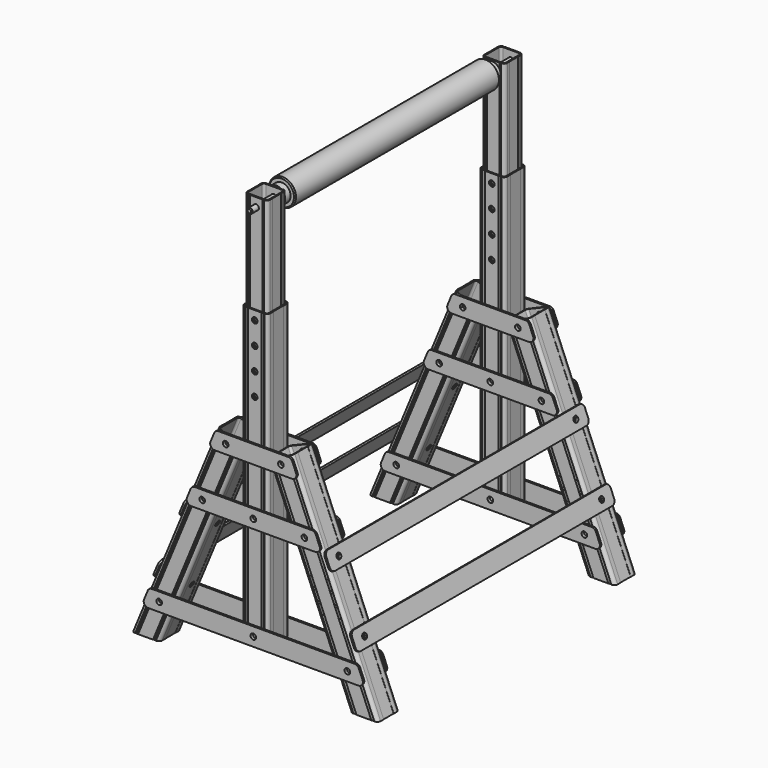
from build123d import *

# Parameters (mm, degrees)
F0_R      = 6.25
F1_DEPTH  = 60
F2_R      = 6.25
F3_DEPTH  = 57.7
F4_R      = 7.5
F6_REACH  = 575.042655099
F7_W      = 57.7
F7_H      = 653.6524637726
F7_R      = 6.25
F8_DEPTH  = 60
F9_R      = 7.5
F11_DEPTH = 653.6524637726
F15_W     = 51
F15_H     = 610
F15_R     = 6.25
F16_DEPTH = 26.15
F17_R     = 7.5
F19_DEPTH = 610
F21_R     = 6.25
F22_DEPTH = 4
F23_R     = 10
F23_2_R   = 10
F23_3_R   = 10
F27_W     = 720
F27_H     = 40
F27_R     = 6.25
F28_DEPTH = 4
F29_R     = 10
F29_2_R   = 10
F32_R     = 5.9
F33_DEPTH = 375
F36_SIZE  = 2
F38_SIZE  = 2.5


# Not quite as in the source:
# - a feature names something its author has since deleted; it is built from what else it names


with BuildPart() as f1:
    # F0 (on Front) → F1 (new body)
    with BuildSketch(Plane.XZ):
        Polygon((-62.4540299569, 0), (0, 0), (-191.3417161825, 461.9397662556), (-244.6495652084, 439.8589322082), align=None)
        with Locations((-64.9222677495, 81.3475362274)):
            Circle(F0_R, mode=Mode.SUBTRACT)
        with Locations((-160.5931258407, 312.3174193552)):
            Circle(F0_R, mode=Mode.SUBTRACT)
        with Locations((-213.0207560747, 438.8889153093)):
            Circle(F0_R, mode=Mode.SUBTRACT)
    extrude(amount=F1_DEPTH)

    # F2 (on face) → F3 (cut, through all)
    with BuildSketch(Plane(origin=(0, 0, 0), x_dir=(0, 1, 0), z_dir=(0.9238795325, 0, 0.3826834324))):
        with Locations((-30, 150)):
            Circle(F2_R)
        with Locations((-30, 300)):
            Circle(F2_R)
    extrude(amount=-F3_DEPTH, mode=Mode.SUBTRACT)

    # F4
    f4_edges = [f1.edges().sort_by_distance(p)[0] for p in [
        (-153.551798, -60, 219.929466),
        (-95.670858, -60, 230.969883),
        (-153.551798, 0, 219.929466),
        (-95.670858, 0, 230.969883),
    ]]
    fillet(f4_edges, radius=F4_R)

    f6_end = f1.faces().sort_by_distance((-31.2270149784, -30, 0))[0]
    # F5 (on face) → F6 (cut, up to a face of the model that its end follows)
    with BuildSketch(Plane(origin=(-191.3417161825, 0, 461.9397662556), x_dir=(0.9238795325, 0, 0.3826834324), z_dir=(-0.3826834324, 0, 0.9238795325))):
        Polygon((-45.2, -59), (-46.2, -60), (-44.2, -60), align=None)
        Polygon((-47.2, -59), (-48.2, -60), (-46.2, -60), align=None)
        Polygon((-49.2, -59), (-50.2, -60), (-48.2, -60), align=None)
        Polygon((-8.5, -59), (-9.5, -60), (-7.5, -60), align=None)
        Polygon((-10.5, -59), (-11.5, -60), (-9.5, -60), align=None)
        Polygon((-12.5, -59), (-13.5, -60), (-11.5, -60), align=None)
        Polygon((-0.3, -44), (0, -44), (0, -16), (-0.3, -16), (-0.3, -30), align=None)
        Polygon((-57.4, -44), (-57.4, -30), (-57.4, -16), (-57.7, -16), (-57.7, -44), align=None)
        Polygon((-48.2, 0), (-50.2, 0), (-49.2, -1), align=None)
        Polygon((-46.2, 0), (-48.2, 0), (-47.2, -1), align=None)
        Polygon((-44.2, 0), (-46.2, 0), (-45.2, -1), align=None)
        Polygon((-7.5, 0), (-9.5, 0), (-8.5, -1), align=None)
        Polygon((-9.5, 0), (-11.5, 0), (-10.5, -1), align=None)
        Polygon((-11.5, 0), (-13.5, 0), (-12.5, -1), align=None)
        with BuildLine():
            Line((-54.8, -30), (-54.8, -52.5))
            ThreePointArc((-54.8, -52.5), (-53.4526911935, -55.7526911935), (-50.2, -57.1))
            Line((-50.2, -57.1), (-28.85, -57.1))
            Line((-28.85, -57.1), (-7.5, -57.1))
            ThreePointArc((-7.5, -57.1), (-4.2473088065, -55.7526911935), (-2.9, -52.5))
            Line((-2.9, -52.5), (-2.9, -30))
            Line((-2.9, -30), (-2.9, -7.5))
            ThreePointArc((-2.9, -7.5), (-4.2473088065, -4.2473088065), (-7.5, -2.9))
            Line((-7.5, -2.9), (-28.85, -2.9))
            Line((-28.85, -2.9), (-50.2, -2.9))
            ThreePointArc((-50.2, -2.9), (-53.4526911935, -4.2473088065), (-54.8, -7.5))
            Line((-54.8, -7.5), (-54.8, -30))
        make_face()
    f6_long = extrude(amount=-F6_REACH, mode=Mode.PRIVATE)
    add(split(f6_long, bisect_by=f6_end, keep=Keep.BOTTOM, mode=Mode.PRIVATE), mode=Mode.SUBTRACT)


with BuildPart() as f8:
    # F7 (on face) → F8 (new body)
    with BuildSketch(Plane.XZ.offset(60)):
        with Locations((-274.4995652084, 393.1737681137)):
            Rectangle(F7_W, F7_H)
        with Locations((-274.4995652084, 81.3475362274)):
            Circle(F7_R, mode=Mode.SUBTRACT)
        with Locations((-274.4995652084, 312.3174193552)):
            Circle(F7_R, mode=Mode.SUBTRACT)
        with Locations((-274.4995652084, 600)):
            Circle(F7_R, mode=Mode.SUBTRACT)
        with Locations((-274.4995652084, 650)):
            Circle(F7_R, mode=Mode.SUBTRACT)
        with Locations((-274.4995652084, 700)):
            Circle(F7_R, mode=Mode.SUBTRACT)
        with Locations((-274.4995652084, 550)):
            Circle(F7_R, mode=Mode.SUBTRACT)
    extrude(amount=-F8_DEPTH)

    # F9
    f9_edges = [f8.edges().sort_by_distance(p)[0] for p in [
        (-303.349565, 0, 393.173768),
        (-303.349565, -60, 393.173768),
        (-245.649565, -60, 393.173768),
        (-245.649565, 0, 393.173768),
    ]]
    fillet(f9_edges, radius=F9_R)

    # F10 (on face) → F11 (cut, through all)
    with BuildSketch(Plane.XY.offset(720)):
        Polygon((-290.8495652084, -59), (-291.8495652084, -60), (-289.8495652084, -60), align=None)
        Polygon((-292.8495652084, -59), (-293.8495652084, -60), (-291.8495652084, -60), align=None)
        Polygon((-294.8495652084, -59), (-295.8495652084, -60), (-293.8495652084, -60), align=None)
        Polygon((-303.3495652084, -16), (-303.3495652084, -44), (-303.0495652084, -44), (-303.0495652084, -30), (-303.0495652084, -16), align=None)
        Polygon((-254.1495652084, -59), (-255.1495652084, -60), (-253.1495652084, -60), align=None)
        Polygon((-256.1495652084, -59), (-257.1495652084, -60), (-255.1495652084, -60), align=None)
        Polygon((-258.1495652084, -59), (-259.1495652084, -60), (-257.1495652084, -60), align=None)
        Polygon((-245.9495652084, -44), (-245.6495652084, -44), (-245.6495652084, -16), (-245.9495652084, -16), (-245.9495652084, -30), align=None)
        Polygon((-253.1495652084, 0), (-255.1495652084, 0), (-254.1495652084, -1), align=None)
        Polygon((-255.1495652084, 0), (-257.1495652084, 0), (-256.1495652084, -1), align=None)
        Polygon((-257.1495652084, 0), (-259.1495652084, 0), (-258.1495652084, -1), align=None)
        Polygon((-293.8495652084, 0), (-295.8495652084, 0), (-294.8495652084, -1), align=None)
        Polygon((-291.8495652084, 0), (-293.8495652084, 0), (-292.8495652084, -1), align=None)
        Polygon((-289.8495652084, 0), (-291.8495652084, 0), (-290.8495652084, -1), align=None)
        with BuildLine():
            Line((-300.4495652084, -30), (-300.4495652084, -52.5))
            ThreePointArc((-300.4495652084, -52.5), (-299.1022564019, -55.7526911935), (-295.8495652084, -57.1))
            Line((-295.8495652084, -57.1), (-274.4995652084, -57.1))
            Line((-274.4995652084, -57.1), (-253.1495652084, -57.1))
            ThreePointArc((-253.1495652084, -57.1), (-249.896874015, -55.7526911935), (-248.5495652084, -52.5))
            Line((-248.5495652084, -52.5), (-248.5495652084, -30))
            Line((-248.5495652084, -30), (-248.5495652084, -7.5))
            ThreePointArc((-248.5495652084, -7.5), (-249.896874015, -4.2473088065), (-253.1495652084, -2.9))
            Line((-253.1495652084, -2.9), (-274.4995652084, -2.9))
            Line((-274.4995652084, -2.9), (-295.8495652084, -2.9))
            ThreePointArc((-295.8495652084, -2.9), (-299.1022564019, -4.2473088065), (-300.4495652084, -7.5))
            Line((-300.4495652084, -7.5), (-300.4495652084, -30))
        make_face()
    extrude(amount=-F11_DEPTH, mode=Mode.SUBTRACT)


with BuildPart() as f16:
    # F15 (on mid) → F16 (new body, symmetric)
    with BuildSketch(Plane(origin=(0, -30, 0), x_dir=(-1, 0, 0), z_dir=(0, 1, 0))):
        with Locations((274.4995652084, 635)):
            Rectangle(F15_W, F15_H)
        with Locations((274.4995652084, 350)):
            Circle(F15_R, mode=Mode.SUBTRACT)
        with Locations((274.4995652084, 400)):
            Circle(F15_R, mode=Mode.SUBTRACT)
        with Locations((274.4995652084, 450)):
            Circle(F15_R, mode=Mode.SUBTRACT)
        with Locations((274.4995652084, 500)):
            Circle(F15_R, mode=Mode.SUBTRACT)
        with Locations((274.4995652084, 550)):
            Circle(F15_R, mode=Mode.SUBTRACT)
        with Locations((274.4995652084, 600)):
            Circle(F15_R, mode=Mode.SUBTRACT)
        with Locations((274.4995652084, 650)):
            Circle(F15_R, mode=Mode.SUBTRACT)
        with Locations((274.4995652084, 700)):
            Circle(F15_R, mode=Mode.SUBTRACT)
        with Locations((274.4995652084, 920)):
            Circle(F15_R, mode=Mode.SUBTRACT)
    extrude(amount=F16_DEPTH, both=True)

    # F17
    f17_edges = [f16.edges().sort_by_distance(p)[0] for p in [
        (-248.999565, -56.15, 635),
        (-299.999565, -56.15, 635),
        (-248.999565, -3.85, 635),
        (-299.999565, -3.85, 635),
    ]]
    fillet(f17_edges, radius=F17_R)

    # F18 (on face) → F19 (cut, through all)
    with BuildSketch(Plane.XY.offset(940)):
        Polygon((-248.9995652084, -42.15), (-248.9995652084, -17.85), (-249.2495652084, -17.85), (-249.2495652084, -30), (-249.2495652084, -42.15), align=None)
        Polygon((-299.7495652084, -17.85), (-299.9995652084, -17.85), (-299.9995652084, -42.15), (-299.7495652084, -42.15), (-299.7495652084, -30), align=None)
        Polygon((-292.4995652084, -56.15), (-290.4995652084, -56.15), (-291.4995652084, -55.15), align=None)
        Polygon((-290.4995652084, -56.15), (-288.4995652084, -56.15), (-289.4995652084, -55.15), align=None)
        Polygon((-258.4995652084, -56.15), (-256.4995652084, -56.15), (-257.4995652084, -55.15), align=None)
        Polygon((-260.4995652084, -56.15), (-258.4995652084, -56.15), (-259.4995652084, -55.15), align=None)
        Polygon((-257.4995652084, -4.85), (-256.4995652084, -3.85), (-258.4995652084, -3.85), align=None)
        Polygon((-259.4995652084, -4.85), (-258.4995652084, -3.85), (-260.4995652084, -3.85), align=None)
        Polygon((-291.4995652084, -4.85), (-290.4995652084, -3.85), (-292.4995652084, -3.85), align=None)
        Polygon((-289.4995652084, -4.85), (-288.4995652084, -3.85), (-290.4995652084, -3.85), align=None)
        with BuildLine():
            Line((-251.8995652084, -30), (-251.8995652084, -11.35))
            ThreePointArc((-251.8995652084, -11.35), (-253.246874015, -8.0973088065), (-256.4995652084, -6.75))
            Line((-256.4995652084, -6.75), (-274.4995652084, -6.75))
            Line((-274.4995652084, -6.75), (-292.4995652084, -6.75))
            ThreePointArc((-292.4995652084, -6.75), (-295.7522564019, -8.0973088065), (-297.0995652084, -11.35))
            Line((-297.0995652084, -11.35), (-297.0995652084, -30))
            Line((-297.0995652084, -30), (-297.0995652084, -48.65))
            ThreePointArc((-297.0995652084, -48.65), (-295.7522564019, -51.9026911935), (-292.4995652084, -53.25))
            Line((-292.4995652084, -53.25), (-274.4995652084, -53.25))
            Line((-274.4995652084, -53.25), (-256.4995652084, -53.25))
            ThreePointArc((-256.4995652084, -53.25), (-253.246874015, -51.9026911935), (-251.8995652084, -48.65))
            Line((-251.8995652084, -48.65), (-251.8995652084, -30))
        make_face()
    extrude(amount=-F19_DEPTH, mode=Mode.SUBTRACT)


with BuildPart() as f20_1:
    # F20: instance of F1
    add(f1.part.mirror(Plane(origin=(-274.4995652084, -30, 393.1737681137), x_dir=(0, 1, 0), z_dir=(1, 0, 0))))


with BuildPart() as f22:
    # F21 (on face) → F22 (new body)
    with BuildSketch(Plane.XZ.offset(60)):
        Polygon((-137.6503821098, 332.3174193552), (-411.3487483071, 332.3174193552), (-427.9172908021, 292.3174193552), (-121.0818396148, 292.3174193552), align=None)
        with Locations((-388.4060045762, 312.3174193552)):
            Circle(F21_R, mode=Mode.SUBTRACT)
        with Locations((-274.4995652084, 312.3174193552)):
            Circle(F21_R, mode=Mode.SUBTRACT)
        with Locations((-160.5931258407, 312.3174193552)):
            Circle(F21_R, mode=Mode.SUBTRACT)
    extrude(amount=F22_DEPTH)

    # F23
    f23_edges = [f22.edges().sort_by_distance(p)[0] for p in [
        (-137.650382, -62, 332.317419),
        (-121.08184, -62, 292.317419),
        (-427.917291, -62, 292.317419),
        (-411.348748, -62, 332.317419),
    ]]
    fillet(f23_edges, radius=F23_R)


with BuildPart() as f22b:
    # F21 (on face) → F22, piece 2 (new body)
    with BuildSketch(Plane.XZ.offset(60)):
        Polygon((-41.9795240185, 101.3475362274), (-507.0196063984, 101.3475362274), (-523.5881488933, 61.3475362274), (-25.4109815236, 61.3475362274), align=None)
        with Locations((-484.0768626674, 81.3475362274)):
            Circle(F21_R, mode=Mode.SUBTRACT)
        with Locations((-274.4995652084, 81.3475362274)):
            Circle(F21_R, mode=Mode.SUBTRACT)
        with Locations((-64.9222677495, 81.3475362274)):
            Circle(F21_R, mode=Mode.SUBTRACT)
    extrude(amount=F22_DEPTH)

    # F23#2
    f23_2_edges = [f22b.edges().sort_by_distance(p)[0] for p in [
        (-523.588149, -62, 61.347536),
        (-507.019606, -62, 101.347536),
        (-25.410982, -62, 61.347536),
        (-41.979524, -62, 101.347536),
    ]]
    fillet(f23_2_edges, radius=F23_2_R)


with BuildPart() as f22c:
    # F21 (on face) → F22, piece 3 (new body)
    with BuildSketch(Plane.XZ.offset(60)):
        Polygon((-190.0780123438, 458.8889153093), (-358.9211180731, 458.8889153093), (-375.489660568, 418.8889153093), (-173.5094698489, 418.8889153093), align=None)
        with Locations((-335.9783743421, 438.8889153093)):
            Circle(F21_R, mode=Mode.SUBTRACT)
        with Locations((-213.0207560747, 438.8889153093)):
            Circle(F21_R, mode=Mode.SUBTRACT)
    extrude(amount=F22_DEPTH)

    # F23#3
    f23_3_edges = [f22c.edges().sort_by_distance(p)[0] for p in [
        (-358.921118, -62, 458.888915),
        (-375.489661, -62, 418.888915),
        (-190.078012, -62, 458.888915),
        (-173.50947, -62, 418.888915),
    ]]
    fillet(f23_3_edges, radius=F23_3_R)


with BuildPart() as f24_1:
    # F24: instance of F22b
    add(f22b.part.mirror(Plane(origin=(-274.4995652084, -30, 390.7594579348), x_dir=(-1, 0, 0), z_dir=(0, 1, 0))))


with BuildPart() as f24_2:
    # F24: instance of F22
    add(f22.part.mirror(Plane(origin=(-274.4995652084, -30, 390.7594579348), x_dir=(-1, 0, 0), z_dir=(0, 1, 0))))


with BuildPart() as f24_3:
    # F24: instance of F22c
    add(f22c.part.mirror(Plane(origin=(-274.4995652084, -30, 390.7594579348), x_dir=(-1, 0, 0), z_dir=(0, 1, 0))))


with BuildPart() as f26_1:
    # F26: instance of F1
    add(f1.part.mirror(Plane(origin=(-274.4995652084, -360, 389.7798079408), x_dir=(1, 0, 0), z_dir=(0, -1, 0))))


with BuildPart() as f26_2:
    # F26: instance of F20_1
    add(f20_1.part.mirror(Plane(origin=(-274.4995652084, -360, 389.7798079408), x_dir=(1, 0, 0), z_dir=(0, -1, 0))))


with BuildPart() as f26_3:
    # F26: instance of F22b
    add(f22b.part.mirror(Plane(origin=(-274.4995652084, -360, 389.7798079408), x_dir=(1, 0, 0), z_dir=(0, -1, 0))))


with BuildPart() as f26_4:
    # F26: instance of F22
    add(f22.part.mirror(Plane(origin=(-274.4995652084, -360, 389.7798079408), x_dir=(1, 0, 0), z_dir=(0, -1, 0))))


with BuildPart() as f26_5:
    # F26: instance of F22c
    add(f22c.part.mirror(Plane(origin=(-274.4995652084, -360, 389.7798079408), x_dir=(1, 0, 0), z_dir=(0, -1, 0))))


with BuildPart() as f26_6:
    # F26: instance of F24_2
    add(f24_2.part.mirror(Plane(origin=(-274.4995652084, -360, 389.7798079408), x_dir=(1, 0, 0), z_dir=(0, -1, 0))))


with BuildPart() as f26_7:
    # F26: instance of F24_3
    add(f24_3.part.mirror(Plane(origin=(-274.4995652084, -360, 389.7798079408), x_dir=(1, 0, 0), z_dir=(0, -1, 0))))


with BuildPart() as f26_8:
    # F26: instance of F24_1
    add(f24_1.part.mirror(Plane(origin=(-274.4995652084, -360, 389.7798079408), x_dir=(1, 0, 0), z_dir=(0, -1, 0))))


with BuildPart() as f26_9:
    # F26: instance of F8
    add(f8.part.mirror(Plane(origin=(-274.4995652084, -360, 389.7798079408), x_dir=(1, 0, 0), z_dir=(0, -1, 0))))


with BuildPart() as f26_10:
    # F26: instance of F16
    add(f16.part.mirror(Plane(origin=(-274.4995652084, -360, 389.7798079408), x_dir=(1, 0, 0), z_dir=(0, -1, 0))))


with BuildPart() as f28:
    # F27 (on face) → F28 (new body)
    with BuildSketch(Plane(origin=(0, 0, 0), x_dir=(0, 1, 0), z_dir=(0.9238795325, 0, 0.3826834324))):
        with Locations((-360, 150)):
            Rectangle(F27_W, F27_H)
        with Locations((-690, 150)):
            Circle(F27_R, mode=Mode.SUBTRACT)
        with Locations((-30, 150)):
            Circle(F27_R, mode=Mode.SUBTRACT)
    extrude(amount=F28_DEPTH)

    # F29
    f29_edges = [f28.edges().sort_by_distance(p)[0] for p in [
        (-63.208424, -720, 157.824887),
        (-47.901087, -720, 120.869706),
        (-63.208424, 0, 157.824887),
        (-47.901087, 0, 120.869706),
    ]]
    fillet(f29_edges, radius=F29_R)


with BuildPart() as f28b:
    # F27 (on face) → F28, piece 2 (new body)
    with BuildSketch(Plane(origin=(0, 0, 0), x_dir=(0, 1, 0), z_dir=(0.9238795325, 0, 0.3826834324))):
        with Locations((-360, 300)):
            Rectangle(F27_W, F27_H)
        with Locations((-690, 300)):
            Circle(F27_R, mode=Mode.SUBTRACT)
        with Locations((-30, 300)):
            Circle(F27_R, mode=Mode.SUBTRACT)
    extrude(amount=F28_DEPTH)

    # F29#2
    f29_2_edges = [f28b.edges().sort_by_distance(p)[0] for p in [
        (-120.610939, -720, 296.406817),
        (-105.303602, -720, 259.451636),
        (-105.303602, 0, 259.451636),
        (-120.610939, 0, 296.406817),
    ]]
    fillet(f29_2_edges, radius=F29_2_R)


with BuildPart() as f31_1:
    # F31: instance of F28
    add(f28.part.mirror(Plane(origin=(-274.4995652084, -30, 635), x_dir=(0, -1, 0), z_dir=(-1, 0, 0))))


with BuildPart() as f31_2:
    # F31: instance of F28b
    add(f28b.part.mirror(Plane(origin=(-274.4995652084, -30, 635), x_dir=(0, -1, 0), z_dir=(-1, 0, 0))))


with BuildPart() as f33:
    # F32 (on offset) → F33 (new body, symmetric)
    with BuildSketch(Plane.XZ.offset(360)):
        with Locations((-274.4995652084, 920)):
            Circle(F32_R)
    extrude(amount=F33_DEPTH, both=True)

    # F36
    f36_edges = [f33.edges().sort_by_distance(p)[0] for p in [
        (-280.399565, -735, 920),
        (-280.399565, 15, 920),
    ]]
    chamfer(f36_edges, length=F36_SIZE)


with BuildPart() as f35:
    # F34 (on mid) → F35 (revolve)
    with BuildSketch(Plane(origin=(-274.4995652084, 0, 0), x_dir=(0, -1, 0), z_dir=(-1, 0, 0))):
        Polygon((60, 940), (60, 926.25), (360, 926.25), (660, 926.25), (660, 940), (645, 940), (645, 950), (360, 950), (75, 950), (75, 940), align=None)
    revolve(axis=Axis((-274.4995652084, -360, 920), (0, -1, 0)))

    # F38
    f38_edges = [f35.edges().sort_by_distance(p)[0] for p in [
        (-274.499565, -645, 890),
        (-274.499565, -75, 890),
    ]]
    chamfer(f38_edges, length=F38_SIZE)


solid = Compound([f1.part, f8.part, f16.part, f20_1.part, f22.part, f22b.part, f22c.part, f24_1.part, f24_2.part, f24_3.part, f26_1.part, f26_2.part, f26_3.part, f26_4.part, f26_5.part, f26_6.part, f26_7.part, f26_8.part, f26_9.part, f26_10.part, f28.part, f28b.part, f31_1.part, f31_2.part, f33.part, f35.part])
